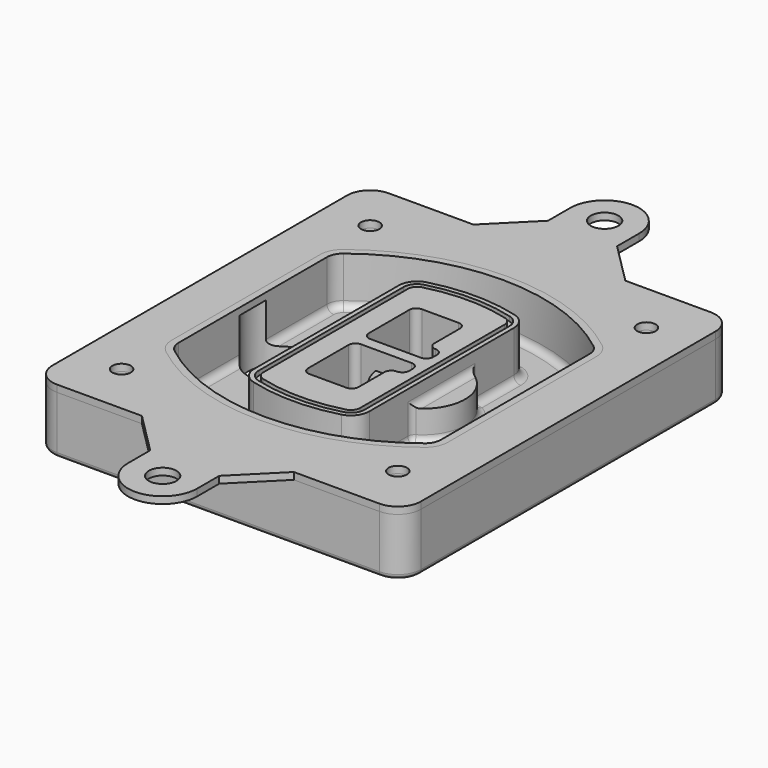
from build123d import *

# Parameters (mm, degrees)
F0_R      = 4
F1_DEPTH  = 25
F2_DEPTH  = 3
F3_DEPTH  = 18
F5_DEPTH  = 21
F6_DEPTH  = 2
F8_DEPTH  = 20
F9_DEPTH  = 16
F10_DEPTH = 25
F7_R      = 6
F7_R_2    = 4
F11_DEPTH = 6
F13_DEPTH = 9
F14_R     = 3
F15_R     = 2
F16_R     = 6
F16_R_2   = 4
F17_DEPTH = 3


# Not quite as in the source:
# - a feature names something its author has since deleted; it is built from what else it names


with BuildPart() as f1:
    # F0 (on Top) → F1 (new body)
    with BuildSketch(Plane.XY):
        with BuildLine():
            ThreePointArc((-80, -80), (-77.0710678119, -87.0710678119), (-70, -90))
            Line((-70, -90), (70, -90))
            ThreePointArc((70, -90), (77.0710678119, -87.0710678119), (80, -80))
            Line((80, -80), (80, 80))
            ThreePointArc((80, 80), (77.0710678119, 87.0710678119), (70, 90))
            Line((70, 90), (-70, 90))
            ThreePointArc((-70, 90), (-77.0710678119, 87.0710678119), (-80, 80))
            Line((-80, 80), (-80, -80))
        make_face()
        with Locations((-60, -67.5)):
            Circle(F0_R, mode=Mode.SUBTRACT)
        with Locations((60, -67.5)):
            Circle(F0_R, mode=Mode.SUBTRACT)
        with Locations((-60, 67.5)):
            Circle(F0_R, mode=Mode.SUBTRACT)
        with BuildLine():
            ThreePointArc((-64, 40.2934422872), (-62.5820384798, 46.4328484224), (-58.6153846154, 51.3286200352))
            ThreePointArc((-58.6153846154, 51.3286200352), (0, 71.5), (58.6153846154, 51.3286200352))
            ThreePointArc((58.6153846154, 51.3286200352), (62.5820384798, 46.4328484224), (64, 40.2934422872))
            Line((64, 40.2934422872), (64, -40.2934422872))
            ThreePointArc((64, -40.2934422872), (62.5820384798, -46.4328484224), (58.6153846154, -51.3286200352))
            ThreePointArc((58.6153846154, -51.3286200352), (0, -71.5), (-58.6153846154, -51.3286200352))
            ThreePointArc((-58.6153846154, -51.3286200352), (-62.5820384798, -46.4328484224), (-64, -40.2934422872))
            Line((-64, -40.2934422872), (-64, 40.2934422872))
        make_face(mode=Mode.SUBTRACT)
        with Locations((60, 67.5)):
            Circle(F0_R, mode=Mode.SUBTRACT)
        with BuildLine():
            ThreePointArc((58.6153846154, 51.3286200352), (0, 71.5), (-58.6153846154, 51.3286200352))
            ThreePointArc((-58.6153846154, 51.3286200352), (-62.5820384798, 46.4328484224), (-64, 40.2934422872))
            Line((-64, 40.2934422872), (-64, -40.2934422872))
            ThreePointArc((-64, -40.2934422872), (-62.5820384798, -46.4328484224), (-58.6153846154, -51.3286200352))
            ThreePointArc((-58.6153846154, -51.3286200352), (0, -71.5), (58.6153846154, -51.3286200352))
            ThreePointArc((58.6153846154, -51.3286200352), (62.5820384798, -46.4328484224), (64, -40.2934422872))
            Line((64, -40.2934422872), (64, 40.2934422872))
            ThreePointArc((64, 40.2934422872), (62.5820384798, 46.4328484224), (58.6153846154, 51.3286200352))
        make_face()
        with BuildLine():
            Line((-60, -40.2934422872), (-60, 40.2934422872))
            ThreePointArc((-60, 40.2934422872), (-58.9871703427, 44.6787323838), (-56.1538461538, 48.1757121072))
            ThreePointArc((-56.1538461538, 48.1757121072), (0, 67.5), (56.1538461538, 48.1757121072))
            ThreePointArc((56.1538461538, 48.1757121072), (58.9871703427, 44.6787323838), (60, 40.2934422872))
            Line((60, 40.2934422872), (60, -40.2934422872))
            ThreePointArc((60, -40.2934422872), (58.9871703427, -44.6787323838), (56.1538461538, -48.1757121072))
            ThreePointArc((56.1538461538, -48.1757121072), (0, -67.5), (-56.1538461538, -48.1757121072))
            ThreePointArc((-56.1538461538, -48.1757121072), (-58.9871703427, -44.6787323838), (-60, -40.2934422872))
        make_face(mode=Mode.SUBTRACT)
        with BuildLine():
            ThreePointArc((-56.1538461538, 48.1757121072), (-58.9871703427, 44.6787323838), (-60, 40.2934422872))
            Line((-60, 40.2934422872), (-60, -40.2934422872))
            ThreePointArc((-60, -40.2934422872), (-58.9871703427, -44.6787323838), (-56.1538461538, -48.1757121072))
            ThreePointArc((-56.1538461538, -48.1757121072), (0, -67.5), (56.1538461538, -48.1757121072))
            ThreePointArc((56.1538461538, -48.1757121072), (58.9871703427, -44.6787323838), (60, -40.2934422872))
            Line((60, -40.2934422872), (60, 40.2934422872))
            ThreePointArc((60, 40.2934422872), (58.9871703427, 44.6787323838), (56.1538461538, 48.1757121072))
            ThreePointArc((56.1538461538, 48.1757121072), (0, 67.5), (-56.1538461538, 48.1757121072))
        make_face()
        with BuildLine():
            ThreePointArc((54.3076923077, 45.8110311612), (56.2910192399, 43.3631453548), (57, 40.2934422872))
            Line((57, 40.2934422872), (57, -40.2934422872))
            ThreePointArc((57, -40.2934422872), (56.2910192399, -43.3631453548), (54.3076923077, -45.8110311612))
            ThreePointArc((54.3076923077, -45.8110311612), (0, -64.5), (-54.3076923077, -45.8110311612))
            ThreePointArc((-54.3076923077, -45.8110311612), (-56.2910192399, -43.3631453548), (-57, -40.2934422872))
            Line((-57, -40.2934422872), (-57, 40.2934422872))
            ThreePointArc((-57, 40.2934422872), (-56.2910192399, 43.3631453548), (-54.3076923077, 45.8110311612))
            ThreePointArc((-54.3076923077, 45.8110311612), (0, 64.5), (54.3076923077, 45.8110311612))
        make_face(mode=Mode.SUBTRACT)
        with BuildLine():
            Line((57, -40.2934422872), (57, 40.2934422872))
            ThreePointArc((57, 40.2934422872), (56.2910192399, 43.3631453548), (54.3076923077, 45.8110311612))
            ThreePointArc((54.3076923077, 45.8110311612), (0, 64.5), (-54.3076923077, 45.8110311612))
            ThreePointArc((-54.3076923077, 45.8110311612), (-56.2910192399, 43.3631453548), (-57, 40.2934422872))
            Line((-57, 40.2934422872), (-57, -40.2934422872))
            ThreePointArc((-57, -40.2934422872), (-56.2910192399, -43.3631453548), (-54.3076923077, -45.8110311612))
            ThreePointArc((-54.3076923077, -45.8110311612), (0, -64.5), (54.3076923077, -45.8110311612))
            ThreePointArc((54.3076923077, -45.8110311612), (56.2910192399, -43.3631453548), (57, -40.2934422872))
        make_face()
    extrude(amount=-F1_DEPTH)

    # F0 (on Top) → F2 (join)
    with BuildSketch(Plane.XY):
        with BuildLine():
            ThreePointArc((-56.1538461538, 48.1757121072), (-58.9871703427, 44.6787323838), (-60, 40.2934422872))
            Line((-60, 40.2934422872), (-60, -40.2934422872))
            ThreePointArc((-60, -40.2934422872), (-58.9871703427, -44.6787323838), (-56.1538461538, -48.1757121072))
            ThreePointArc((-56.1538461538, -48.1757121072), (0, -67.5), (56.1538461538, -48.1757121072))
            ThreePointArc((56.1538461538, -48.1757121072), (58.9871703427, -44.6787323838), (60, -40.2934422872))
            Line((60, -40.2934422872), (60, 40.2934422872))
            ThreePointArc((60, 40.2934422872), (58.9871703427, 44.6787323838), (56.1538461538, 48.1757121072))
            ThreePointArc((56.1538461538, 48.1757121072), (0, 67.5), (-56.1538461538, 48.1757121072))
        make_face()
        with BuildLine():
            ThreePointArc((54.3076923077, 45.8110311612), (56.2910192399, 43.3631453548), (57, 40.2934422872))
            Line((57, 40.2934422872), (57, -40.2934422872))
            ThreePointArc((57, -40.2934422872), (56.2910192399, -43.3631453548), (54.3076923077, -45.8110311612))
            ThreePointArc((54.3076923077, -45.8110311612), (0, -64.5), (-54.3076923077, -45.8110311612))
            ThreePointArc((-54.3076923077, -45.8110311612), (-56.2910192399, -43.3631453548), (-57, -40.2934422872))
            Line((-57, -40.2934422872), (-57, 40.2934422872))
            ThreePointArc((-57, 40.2934422872), (-56.2910192399, 43.3631453548), (-54.3076923077, 45.8110311612))
            ThreePointArc((-54.3076923077, 45.8110311612), (0, 64.5), (54.3076923077, 45.8110311612))
        make_face(mode=Mode.SUBTRACT)
    extrude(amount=F2_DEPTH)

    # F0 (on Top) → F3 (cut)
    with BuildSketch(Plane.XY):
        with BuildLine():
            Line((57, -40.2934422872), (57, 40.2934422872))
            ThreePointArc((57, 40.2934422872), (56.2910192399, 43.3631453548), (54.3076923077, 45.8110311612))
            ThreePointArc((54.3076923077, 45.8110311612), (0, 64.5), (-54.3076923077, 45.8110311612))
            ThreePointArc((-54.3076923077, 45.8110311612), (-56.2910192399, 43.3631453548), (-57, 40.2934422872))
            Line((-57, 40.2934422872), (-57, -40.2934422872))
            ThreePointArc((-57, -40.2934422872), (-56.2910192399, -43.3631453548), (-54.3076923077, -45.8110311612))
            ThreePointArc((-54.3076923077, -45.8110311612), (0, -64.5), (54.3076923077, -45.8110311612))
            ThreePointArc((54.3076923077, -45.8110311612), (56.2910192399, -43.3631453548), (57, -40.2934422872))
        make_face()
    extrude(amount=-F3_DEPTH, mode=Mode.SUBTRACT)

    # F4 (on face) → F5 (join, through all)
    with BuildSketch(Plane.XY.offset(3)):
        with BuildLine():
            ThreePointArc((-25, -39.2465276821), (-23.3511545998, -44.1109737193), (-19.0842911877, -46.9702398883))
            ThreePointArc((-19.0842911877, -46.9702398883), (0, -49.5), (19.0842911877, -46.9702398883))
            ThreePointArc((19.0842911877, -46.9702398883), (23.3511545998, -44.1109737193), (25, -39.2465276821))
            Line((25, -39.2465276821), (25, 39.2465276821))
            ThreePointArc((25, 39.2465276821), (23.3511545998, 44.1109737193), (19.0842911877, 46.9702398883))
            ThreePointArc((19.0842911877, 46.9702398883), (0, 49.5), (-19.0842911877, 46.9702398883))
            ThreePointArc((-19.0842911877, 46.9702398883), (-23.3511545998, 44.1109737193), (-25, 39.2465276821))
            Line((-25, 39.2465276821), (-25, -39.2465276821))
        make_face()
        with BuildLine():
            ThreePointArc((18.5632183908, 45.0393118368), (21.7633659499, 42.89486221), (23, 39.2465276821))
            Line((23, 39.2465276821), (23, -39.2465276821))
            ThreePointArc((23, -39.2465276821), (21.7633659499, -42.89486221), (18.5632183908, -45.0393118368))
            ThreePointArc((18.5632183908, -45.0393118368), (0, -47.5), (-18.5632183908, -45.0393118368))
            ThreePointArc((-18.5632183908, -45.0393118368), (-21.7633659499, -42.89486221), (-23, -39.2465276821))
            Line((-23, -39.2465276821), (-23, 39.2465276821))
            ThreePointArc((-23, 39.2465276821), (-21.7633659499, 42.89486221), (-18.5632183908, 45.0393118368))
            ThreePointArc((-18.5632183908, 45.0393118368), (0, 47.5), (18.5632183908, 45.0393118368))
        make_face(mode=Mode.SUBTRACT)
        with BuildLine():
            Line((23, -39.2465276821), (23, 39.2465276821))
            ThreePointArc((23, 39.2465276821), (21.7633659499, 42.89486221), (18.5632183908, 45.0393118368))
            ThreePointArc((18.5632183908, 45.0393118368), (0, 47.5), (-18.5632183908, 45.0393118368))
            ThreePointArc((-18.5632183908, 45.0393118368), (-21.7633659499, 42.89486221), (-23, 39.2465276821))
            Line((-23, 39.2465276821), (-23, -39.2465276821))
            ThreePointArc((-23, -39.2465276821), (-21.7633659499, -42.89486221), (-18.5632183908, -45.0393118368))
            ThreePointArc((-18.5632183908, -45.0393118368), (0, -47.5), (18.5632183908, -45.0393118368))
            ThreePointArc((18.5632183908, -45.0393118368), (21.7633659499, -42.89486221), (23, -39.2465276821))
        make_face()
        with BuildLine():
            ThreePointArc((18.0421455939, 43.1083837852), (20.1755772999, 41.6787507007), (21, 39.2465276821))
            Line((21, 39.2465276821), (21, -39.2465276821))
            ThreePointArc((21, -39.2465276821), (20.1755772999, -41.6787507007), (18.0421455939, -43.1083837852))
            ThreePointArc((18.0421455939, -43.1083837852), (0, -45.5), (-18.0421455939, -43.1083837852))
            ThreePointArc((-18.0421455939, -43.1083837852), (-20.1755772999, -41.6787507007), (-21, -39.2465276821))
            Line((-21, -39.2465276821), (-21, 39.2465276821))
            ThreePointArc((-21, 39.2465276821), (-20.1755772999, 41.6787507007), (-18.0421455939, 43.1083837852))
            ThreePointArc((-18.0421455939, 43.1083837852), (0, 45.5), (18.0421455939, 43.1083837852))
        make_face(mode=Mode.SUBTRACT)
        with BuildLine():
            Line((21, -39.2465276821), (21, 39.2465276821))
            ThreePointArc((21, 39.2465276821), (20.1755772999, 41.6787507007), (18.0421455939, 43.1083837852))
            ThreePointArc((18.0421455939, 43.1083837852), (0, 45.5), (-18.0421455939, 43.1083837852))
            ThreePointArc((-18.0421455939, 43.1083837852), (-20.1755772999, 41.6787507007), (-21, 39.2465276821))
            Line((-21, 39.2465276821), (-21, -39.2465276821))
            ThreePointArc((-21, -39.2465276821), (-20.1755772999, -41.6787507007), (-18.0421455939, -43.1083837852))
            ThreePointArc((-18.0421455939, -43.1083837852), (0, -45.5), (18.0421455939, -43.1083837852))
            ThreePointArc((18.0421455939, -43.1083837852), (20.1755772999, -41.6787507007), (21, -39.2465276821))
        make_face()
        with BuildLine():
            Line((-8, -2.5), (14, -2.5))
            ThreePointArc((14, -2.5), (16.1213203436, -3.3786796564), (17, -5.5))
            Line((17, -5.5), (17, -7.5))
            ThreePointArc((17, -7.5), (16.1213203436, -9.6213203436), (14, -10.5))
            ThreePointArc((14, -10.5), (11.8786796564, -11.3786796564), (11, -13.5))
            Line((11, -13.5), (11, -27.5))
            ThreePointArc((11, -27.5), (10.1213203436, -29.6213203436), (8, -30.5))
            Line((8, -30.5), (-8, -30.5))
            ThreePointArc((-8, -30.5), (-10.1213203436, -29.6213203436), (-11, -27.5))
            Line((-11, -27.5), (-11, -5.5))
            ThreePointArc((-11, -5.5), (-10.1213203436, -3.3786796564), (-8, -2.5))
        make_face(mode=Mode.SUBTRACT)
        with BuildLine():
            ThreePointArc((-8, 2.5), (-10.1213203436, 3.3786796564), (-11, 5.5))
            Line((-11, 5.5), (-11, 27.5))
            ThreePointArc((-11, 27.5), (-10.1213203436, 29.6213203436), (-8, 30.5))
            Line((-8, 30.5), (8, 30.5))
            ThreePointArc((8, 30.5), (10.1213203436, 29.6213203436), (11, 27.5))
            Line((11, 27.5), (11, 13.5))
            ThreePointArc((11, 13.5), (11.8786796564, 11.3786796564), (14, 10.5))
            ThreePointArc((14, 10.5), (16.1213203436, 9.6213203436), (17, 7.5))
            Line((17, 7.5), (17, 5.5))
            ThreePointArc((17, 5.5), (16.1213203436, 3.3786796564), (14, 2.5))
            Line((14, 2.5), (-8, 2.5))
        make_face(mode=Mode.SUBTRACT)
    extrude(amount=-F5_DEPTH)

    # F4 (on face) → F6 (cut)
    with BuildSketch(Plane.XY.offset(3)):
        with BuildLine():
            Line((23, -39.2465276821), (23, 39.2465276821))
            ThreePointArc((23, 39.2465276821), (21.7633659499, 42.89486221), (18.5632183908, 45.0393118368))
            ThreePointArc((18.5632183908, 45.0393118368), (0, 47.5), (-18.5632183908, 45.0393118368))
            ThreePointArc((-18.5632183908, 45.0393118368), (-21.7633659499, 42.89486221), (-23, 39.2465276821))
            Line((-23, 39.2465276821), (-23, -39.2465276821))
            ThreePointArc((-23, -39.2465276821), (-21.7633659499, -42.89486221), (-18.5632183908, -45.0393118368))
            ThreePointArc((-18.5632183908, -45.0393118368), (0, -47.5), (18.5632183908, -45.0393118368))
            ThreePointArc((18.5632183908, -45.0393118368), (21.7633659499, -42.89486221), (23, -39.2465276821))
        make_face()
        with BuildLine():
            ThreePointArc((18.0421455939, 43.1083837852), (20.1755772999, 41.6787507007), (21, 39.2465276821))
            Line((21, 39.2465276821), (21, -39.2465276821))
            ThreePointArc((21, -39.2465276821), (20.1755772999, -41.6787507007), (18.0421455939, -43.1083837852))
            ThreePointArc((18.0421455939, -43.1083837852), (0, -45.5), (-18.0421455939, -43.1083837852))
            ThreePointArc((-18.0421455939, -43.1083837852), (-20.1755772999, -41.6787507007), (-21, -39.2465276821))
            Line((-21, -39.2465276821), (-21, 39.2465276821))
            ThreePointArc((-21, 39.2465276821), (-20.1755772999, 41.6787507007), (-18.0421455939, 43.1083837852))
            ThreePointArc((-18.0421455939, 43.1083837852), (0, 45.5), (18.0421455939, 43.1083837852))
        make_face(mode=Mode.SUBTRACT)
    extrude(amount=-F6_DEPTH, mode=Mode.SUBTRACT)

    # F7 (on face) → F8 (join)
    with BuildSketch(Plane(origin=(0, 0, -25), x_dir=(1, 0, 0), z_dir=(0, 0, -1))):
        with BuildLine():
            ThreePointArc((3.28842436, 0), (16.7567035675, 13.4682792075), (30.224982775, 0))
            Line((30.224982775, 0), (35.224982775, 0))
            ThreePointArc((35.224982775, 0), (16.7567035675, 18.4682792075), (-1.71157564, 0))
            Line((-1.71157564, 0), (3.28842436, 0))
        make_face()
        with BuildLine():
            Line((3.28842436, 0), (30.224982775, 0))
            ThreePointArc((30.224982775, 0), (16.7567035675, 13.4682792075), (3.28842436, 0))
        make_face()
        with BuildLine():
            ThreePointArc((3.28842436, 0), (16.7567035675, -13.4682792075), (30.224982775, 0))
            Line((30.224982775, 0), (3.28842436, 0))
        make_face()
        with BuildLine():
            Line((35.224982775, 0), (30.224982775, 0))
            ThreePointArc((30.224982775, 0), (16.7567035675, -13.4682792075), (3.28842436, 0))
            Line((3.28842436, 0), (-1.71157564, 0))
            ThreePointArc((-1.71157564, 0), (16.7567035675, -18.4682792075), (35.224982775, 0))
        make_face()
    extrude(amount=-F8_DEPTH)

    # F7 (on face) → F9 (cut)
    with BuildSketch(Plane(origin=(0, 0, -25), x_dir=(1, 0, 0), z_dir=(0, 0, -1))):
        with BuildLine():
            Line((3.28842436, 0), (30.224982775, 0))
            ThreePointArc((30.224982775, 0), (16.7567035675, 13.4682792075), (3.28842436, 0))
        make_face()
        with BuildLine():
            ThreePointArc((3.28842436, 0), (16.7567035675, -13.4682792075), (30.224982775, 0))
            Line((30.224982775, 0), (3.28842436, 0))
        make_face()
    extrude(amount=-F9_DEPTH, mode=Mode.SUBTRACT)

    # F7 (on face) → F10 (cut)
    with BuildSketch(Plane(origin=(0, 0, -25), x_dir=(1, 0, 0), z_dir=(0, 0, -1))):
        with BuildLine():
            Line((-59.0318229325, 0), (-32.0952645175, 0))
            ThreePointArc((-32.0952645175, 0), (-45.563543725, 13.4682792075), (-59.0318229325, 0))
        make_face()
        with BuildLine():
            ThreePointArc((-59.0318229325, 0), (-45.563543725, -13.4682792075), (-32.0952645175, 0))
            Line((-32.0952645175, 0), (-59.0318229325, 0))
        make_face()
    extrude(amount=-F10_DEPTH, mode=Mode.SUBTRACT)

    # F7 (on face) → F11 (cut)
    with BuildSketch(Plane(origin=(0, 0, -25), x_dir=(1, 0, 0), z_dir=(0, 0, -1))):
        with Locations((60, -67.5)):
            Circle(F7_R)
        with Locations((60, -67.5)):
            Circle(F7_R_2, mode=Mode.SUBTRACT)
        with Locations((-60, -67.5)):
            Circle(F7_R)
        with Locations((-60, -67.5)):
            Circle(F7_R_2, mode=Mode.SUBTRACT)
        with Locations((-60, 67.5)):
            Circle(F7_R)
        with Locations((-60, 67.5)):
            Circle(F7_R_2, mode=Mode.SUBTRACT)
        with Locations((60, 67.5)):
            Circle(F7_R)
        with Locations((60, 67.5)):
            Circle(F7_R_2, mode=Mode.SUBTRACT)
    extrude(amount=-F11_DEPTH, mode=Mode.SUBTRACT)

    # F12 (on face) → F13 (cut, through all)
    with BuildSketch(Plane(origin=(0, 0, -9), x_dir=(1, 0, 0), z_dir=(0, 0, -1))):
        with BuildLine():
            Line((11, 13.5), (11, 17.5481537753))
            ThreePointArc((11, 17.5481537753), (2.5696536419, 11.8239143813), (-1.5415842455, 2.5))
            Line((-1.5415842455, 2.5), (3.5224848595, 2.5))
            ThreePointArc((3.5224848595, 2.5), (6.1857188154, 8.3455872281), (11.2536447004, 12.2927168648))
            ThreePointArc((11.2536447004, 12.2927168648), (11.0640958889, 12.8831798879), (11, 13.5))
        make_face()
        with BuildLine():
            ThreePointArc((11.2536447004, -12.2927168648), (6.1857188154, -8.3455872281), (3.5224848595, -2.5))
            Line((3.5224848595, -2.5), (-1.5415842455, -2.5))
            ThreePointArc((-1.5415842455, -2.5), (2.5696536419, -11.8239143813), (11, -17.5481537753))
            Line((11, -17.5481537753), (11, -13.5))
            ThreePointArc((11, -13.5), (11.0640958889, -12.8831798879), (11.2536447004, -12.2927168648))
        make_face()
        with BuildLine():
            ThreePointArc((11.2536447004, 12.2927168648), (6.1857188154, 8.3455872281), (3.5224848595, 2.5))
            Line((3.5224848595, 2.5), (14, 2.5))
            ThreePointArc((14, 2.5), (16.1213203436, 3.3786796564), (17, 5.5))
            Line((17, 5.5), (17, 7.5))
            ThreePointArc((17, 7.5), (16.1213203436, 9.6213203436), (14, 10.5))
            ThreePointArc((14, 10.5), (12.3601599782, 10.9878446101), (11.2536447004, 12.2927168648))
        make_face()
        with BuildLine():
            Line((14, -2.5), (3.5224848595, -2.5))
            ThreePointArc((3.5224848595, -2.5), (6.1857188154, -8.3455872281), (11.2536447004, -12.2927168648))
            ThreePointArc((11.2536447004, -12.2927168648), (12.3601599782, -10.9878446101), (14, -10.5))
            ThreePointArc((14, -10.5), (16.1213203436, -9.6213203436), (17, -7.5))
            Line((17, -7.5), (17, -5.5))
            ThreePointArc((17, -5.5), (16.1213203436, -3.3786796564), (14, -2.5))
        make_face()
    extrude(amount=F13_DEPTH, mode=Mode.SUBTRACT)

    # F14
    f14_edges = [f1.edges().sort_by_distance(p)[0] for p in [
        (-57, -23.703476, -18),
        (-57, 23.703476, -18),
        (25, 0, -5),
        (25, 16.526506, -11.5),
        (25, -16.526506, -11.5),
        (25, -27.886517, -18),
        (35.224983, 0, -18),
    ]]
    fillet(f14_edges, radius=F14_R)

    # F15
    f15_edges = [f1.edges().sort_by_distance(p)[0] for p in [
        (0, -90, -25),
    ]]
    fillet(f15_edges, radius=F15_R)


with BuildPart() as f17:
    # F16 (on face) → F17 (new body, through all)
    with BuildSketch(Plane.XY):
        with BuildLine():
            Line((-15.1517027989, 108), (-33.1517027989, 90))
            Line((-33.1517027989, 90), (32.8331694978, 90))
            Line((32.8331694978, 90), (14.8331694978, 108))
            Line((14.8331694978, 108), (14.8331694978, 108.0777198076))
            Line((14.8331694978, 108.0777198076), (14.8331694978, 120))
            ThreePointArc((14.8331694978, 120), (0.1700044349, 134.9962175973), (-15.1517027989, 120.6735000014))
            Line((-15.1517027989, 120.6735000014), (-15.1517027989, 108.0777198076))
            Line((-15.1517027989, 108.0777198076), (-15.1517027989, 108))
        make_face()
        with Locations((-0.1668305022, 120)):
            Circle(F16_R, mode=Mode.SUBTRACT)
        with BuildLine():
            Line((32.8331694978, 90), (-33.1517027989, 90))
            Line((-33.1517027989, 90), (-70, 90))
            ThreePointArc((-70, 90), (-77.0710678119, 87.0710678119), (-80, 80))
            Line((-80, 80), (-80, -80))
            ThreePointArc((-80, -80), (-77.0710678119, -87.0710678119), (-70, -90))
            Line((-70, -90), (-33.1517027989, -90))
            Line((-33.1517027989, -90), (32.8331694978, -90))
            Line((32.8331694978, -90), (70, -90))
            ThreePointArc((70, -90), (77.0710678119, -87.0710678119), (80, -80))
            Line((80, -80), (80, 80))
            ThreePointArc((80, 80), (77.0710678119, 87.0710678119), (70, 90))
            Line((70, 90), (32.8331694978, 90))
        make_face()
        with Locations((-60, -67.5)):
            Circle(F16_R_2, mode=Mode.SUBTRACT)
        with Locations((60, -67.5)):
            Circle(F16_R_2, mode=Mode.SUBTRACT)
        with Locations((-60, 67.5)):
            Circle(F16_R_2, mode=Mode.SUBTRACT)
        with BuildLine():
            ThreePointArc((-60, 40.2934422872), (-58.9871703427, 44.6787323838), (-56.1538461538, 48.1757121072))
            ThreePointArc((-56.1538461538, 48.1757121072), (0, 67.5), (56.1538461538, 48.1757121072))
            ThreePointArc((56.1538461538, 48.1757121072), (58.9871703427, 44.6787323838), (60, 40.2934422872))
            Line((60, 40.2934422872), (60, -40.2934422872))
            ThreePointArc((60, -40.2934422872), (58.9871703427, -44.6787323838), (56.1538461538, -48.1757121072))
            ThreePointArc((56.1538461538, -48.1757121072), (0, -67.5), (-56.1538461538, -48.1757121072))
            ThreePointArc((-56.1538461538, -48.1757121072), (-58.9871703427, -44.6787323838), (-60, -40.2934422872))
            Line((-60, -40.2934422872), (-60, 40.2934422872))
        make_face(mode=Mode.SUBTRACT)
        with Locations((60, 67.5)):
            Circle(F16_R_2, mode=Mode.SUBTRACT)
        with BuildLine():
            Line((32.8331694978, -90), (-33.1517027989, -90))
            Line((-33.1517027989, -90), (-15.1517027989, -108))
            Line((-15.1517027989, -108), (-15.1517027989, -108.0777198076))
            Line((-15.1517027989, -108.0777198076), (-15.1517027989, -120.6735000014))
            ThreePointArc((-15.1517027989, -120.6735000014), (0.1700044349, -134.9962175973), (14.8331694978, -120))
            Line((14.8331694978, -120), (14.8331694978, -108.0777198076))
            Line((14.8331694978, -108.0777198076), (14.8331694978, -108))
            Line((14.8331694978, -108), (32.8331694978, -90))
        make_face()
        with Locations((-0.1668305022, -120)):
            Circle(F16_R, mode=Mode.SUBTRACT)
    extrude(amount=F17_DEPTH)


solid = Compound([f1.part, f17.part])
